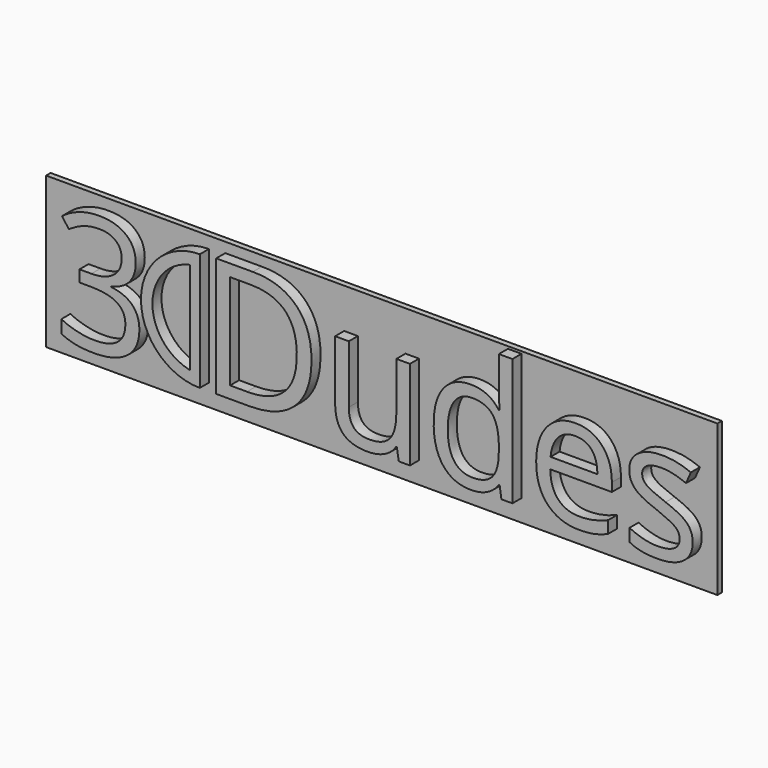
from build123d import *

# Parameters (mm, degrees)
F0_TEXT_SIZE   = 75.0003943124
F0_TEXT_SIZE_2 = 74.9563694828
F1_DEPTH       = 5.08
F2_W           = 301.1126592755
F2_H           = 67.7480641752
F3_DEPTH       = 2.54


# Not quite as in the source:
# - Text() gives the source's letters only with a copy of the font that has no kerning and outlines rounded to 1/6400 em; it was checked with that copy


with BuildPart() as f1:
    # F0 (on Front) → F1 (new body)
    with BuildSketch(Plane.XZ):
        with BuildLine():
            Line((-12.7891199464, -1.8940514427), (-12.7891199464, 24.4979194275))
            ThreePointArc((-12.7891199464, 24.4979194275), (-39.1810908165, -1.8940514427), (-12.7891199464, -28.2860223129))
            Line((-12.7891199464, -28.2860223129), (-12.7891199464, -1.8940514427))
        make_face()
        with BuildLine():
            ThreePointArc((-17.1821049668, -22.6935732825), (-34.0474930298, -1.8940514427), (-17.1821049668, 18.9054703971))
            Line((-17.1821049668, 18.9054703971), (-17.1821049668, -22.6935732825))
        make_face(mode=Mode.SUBTRACT)
        with Locations((-12.7891199464, -28.2656940041)):
            Text('Dudes', F0_TEXT_SIZE, font='Open Sans', text_align=(TextAlign.LEFT, TextAlign.BOTTOM))
        with Locations((-78.3603936434, -29.2628114112)):
            Text('3', F0_TEXT_SIZE_2, font='Open Sans', text_align=(TextAlign.LEFT, TextAlign.BOTTOM))
    extrude(amount=F1_DEPTH)


with BuildPart() as f3:
    # F2 (on Front) → F3 (new body)
    with BuildSketch(Plane.XZ):
        with Locations((64.7545270622, -4.1013201699)):
            Rectangle(F2_W, F2_H)
    extrude(amount=-F3_DEPTH)


solid = Compound([f1.part, f3.part])
